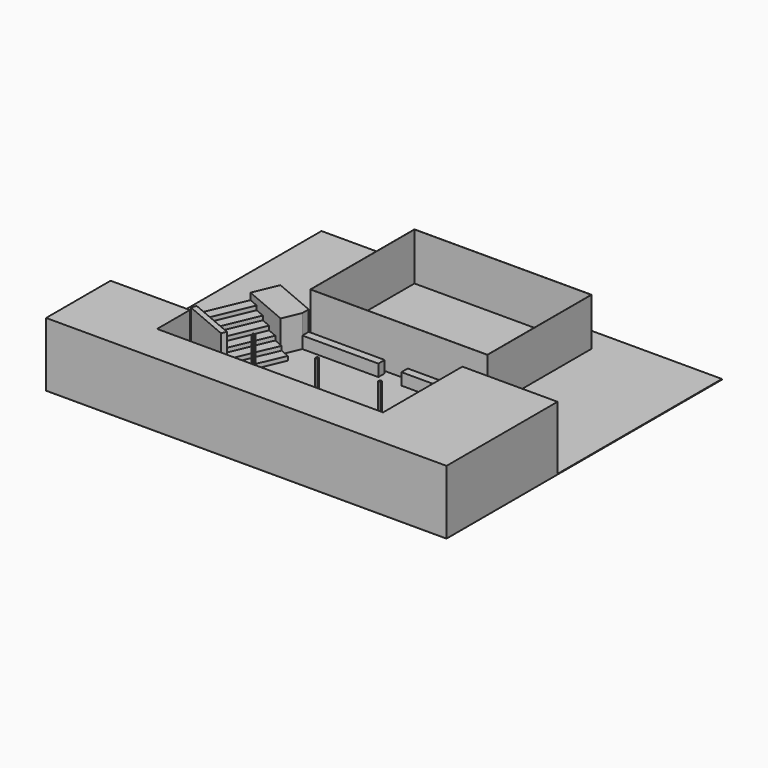
from build123d import *

# Parameters (mm, degrees)
F0_W      = 4191
F0_H      = 304.8
F1_DEPTH  = 457.2
F0_W_2    = 2921
F3_DEPTH  = 2438.4
F2_W      = 84.6666666667
F2_H      = 84.6666666667
F5_DEPTH  = 1219.2
F7_DEPTH  = 1828.8
F8_W      = 15392.4
F8_H      = 13233.4
F9_DEPTH  = 25.4
F10_W     = 6807.2
F10_H     = 5003.8
F10_W_2   = 6797.04
F10_H_2   = 4993.64
F11_DEPTH = 1828.8


with BuildPart() as f1:
    # F0 (on Top) → F1 (new body)
    with BuildSketch(Plane.XY):
        with Locations((2540, 152.4)):
            Rectangle(F0_W, F0_H)
    extrude(amount=F1_DEPTH)


with BuildPart() as f1b:
    # F0 (on Top) → F1, piece 2 (new body)
    with BuildSketch(Plane.XY):
        with Locations((-1905, 152.4)):
            Rectangle(F0_W_2, F0_H)
    extrude(amount=F1_DEPTH)

    # F4 (on Top) → F5 (join)
    with BuildSketch(Plane.XY):
        Polygon((-3655.7759595183, -683.0676722074), (-3365.5, 0), (-3365.5, 304.8), (-5009.0418331298, 1003.2383861683), (-6203.7653557771, -1808.1450191275), (-4660.9, -2463.8), (-4450.5092696668, -2553.2074973917), (-4371.0359386519, -2366.1935148733), (-3950.2544779854, -2545.0085096567), (-3234.9944988518, -861.8826669908), align=None)
    extrude(amount=F5_DEPTH)

    # F6 (on face) → F7 (cut)
    with BuildSketch(Plane(origin=(-805.0836430775, -1894.4958822004, 0), x_dir=(-0.9203444022, 0.3911089125, 0), z_dir=(0.3911089125, 0.9203444022, 0))):
        Polygon((2640.2190854615, 1219.2), (2640.2190854615, 160.8666666667), (3033.9190854615, 160.8666666667), (3033.9190854615, 321.7333333333), (3427.6190854615, 321.7333333333), (3427.6190854615, 482.6), (3821.3190854615, 482.6), (3821.3190854615, 643.4666666667), (4215.0190854615, 643.4666666667), (4215.0190854615, 804.3333333333), (4608.7190854615, 804.3333333333), (4608.7190854615, 965.2), (5002.4190854615, 965.2), (5002.4190854615, 1219.2), align=None)
    extrude(amount=-F7_DEPTH, mode=Mode.SUBTRACT)


with BuildPart() as f3:
    # F2 (on Top) → F3 (new body)
    with BuildSketch(Plane.XY):
        Polygon((4635.5, -1549.4), (4025.9, -1549.4), (4025.9, -5359.4), (-4660.9, -5359.4), (-4660.9, -3784.6), (-7708.9, -3784.6), (-7708.9, -6883.4), (4635.5, -6883.4), (7683.5, -6883.4), (7683.5, -1549.4), align=None)
    extrude(amount=F3_DEPTH)


with BuildPart() as f3b:
    # F2 (on Top) → F3, piece 2 (new body)
    with BuildSketch(Plane.XY):
        with Locations((-2180.1666666667, -3826.9333333333)):
            Rectangle(F2_W, F2_H)
    extrude(amount=F3_DEPTH)


with BuildPart() as f3c:
    # F2 (on Top) → F3, piece 3 (new body)
    with BuildSketch(Plane.XY):
        with Locations((266.7, -3826.9333333333)):
            Rectangle(F2_W, F2_H)
    extrude(amount=F3_DEPTH)


with BuildPart() as f3d:
    # F2 (on Top) → F3, piece 4 (new body)
    with BuildSketch(Plane.XY):
        with Locations((2688.1666666667, -3826.9333333333)):
            Rectangle(F2_W, F2_H)
    extrude(amount=F3_DEPTH)


with BuildPart() as f9:
    # F8 (on Top) → F9 (new body)
    with BuildSketch(Plane.XY):
        with Locations((-12.7, -266.7)):
            Rectangle(F8_W, F8_H)
    extrude(amount=-F9_DEPTH)

    # F10 (on Top) → F11 (join)
    with BuildSketch(Plane.XY):
        with Locations((0, 2933.7)):
            Rectangle(F10_W, F10_H)
        with Locations((0, 2933.7)):
            Rectangle(F10_W_2, F10_H_2, mode=Mode.SUBTRACT)
    extrude(amount=F11_DEPTH)


solid = Compound([f1.part, f1b.part, f3.part, f3b.part, f3c.part, f3d.part, f9.part])
